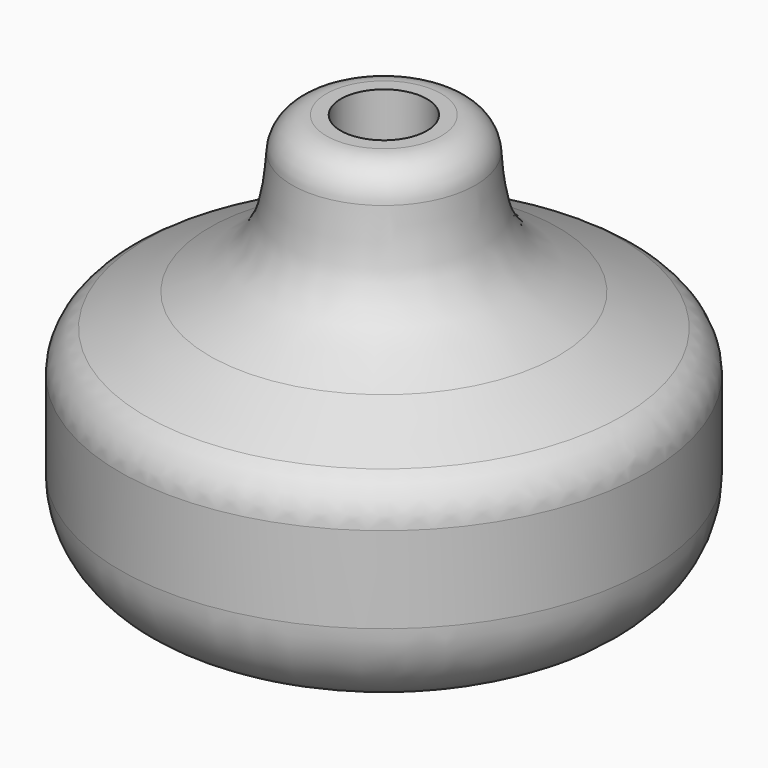
from build123d import *

# Parameters (mm, degrees)
F2_R     = 10.16
F3_R     = 5.08
F4_R     = 4.76885
F5_DEPTH = 11.43
F6_R     = 1.6002
F7_DEPTH = 19.685
F8_R     = 3.81


# Not quite as in the source:
# - a fillet or chamfer that OpenCascade refuses, or shapes differently, is made with other operations: its cross-section is extruded or revolved along the edge and cut away or added


with BuildPart() as f1:
    # F0 (on Front) → F1 (revolve)
    with BuildSketch(Plane.XZ):
        Polygon((0, 54.61), (0, 0), (10.16, 9.5882897328), (29.21, 9.5882897328), (29.21, 32.4482897328), (10.16, 41.9100038707), (10.16, 54.61), align=None)
    revolve(axis=Axis((0, 0, 27.305), (0, 0, 1)))

    # F2
    f2_edges = [f1.edges().sort_by_distance(p)[0] for p in [
        (-29.21, 0, 9.58829),
    ]]
    fillet(f2_edges, radius=F2_R)

    # F3
    f3_edges = [f1.edges().sort_by_distance(p)[0] for p in [
        (-29.21, 0, 32.44829),
    ]]
    fillet(f3_edges, radius=F3_R)

    # F4 (on face) → F5 (cut)
    with BuildSketch(Plane.XY.offset(54.61)):
        Circle(F4_R)
    extrude(amount=-F5_DEPTH, mode=Mode.SUBTRACT)

    # F6 (on Top) → F7 (cut)
    with BuildSketch(Plane.XY):
        Circle(F6_R)
    extrude(amount=F7_DEPTH, mode=Mode.SUBTRACT)

    # F8
    f8_edges = [f1.edges().sort_by_distance(p)[0] for p in [
        (-10.16, 0, 54.61),
    ]]
    fillet(f8_edges, radius=F8_R)

    # F9: fillet of radius 16.51 on 3 edges, made by hand

    # F9_s1 → F9_t2 (revolve)
    with BuildSketch(Plane.XZ):
        with BuildLine():
            add(Edge.make_bspline(
                [(10.1513687758, 51.056311199), (10.7891371387, 41.5975253532), (19.279794422, 37.3804034604)],
                knots=[0, 0, 0, 1, 1, 1], degree=2, weights=[1, 1.8571428571, 1]))
            Line((19.279794422, 37.3804034604), (18.5453771838, 35.9017445003))
            Line((18.5453771838, 35.9017445003), (9.4255827618, 40.4313449106))
            Line((9.4255827618, 40.4313449106), (8.509, 41.9100038707))
            ThreePointArc((8.509, 41.9100038707), (8.509, 50.8), (8.5041089729, 50.9452430127))
            Line((8.5041089729, 50.9452430127), (10.1513687758, 51.056311199))
        make_face()
    revolve(axis=Axis((0, 0, 41.9100038707), (0, 0, 1)))


solid = f1.part
